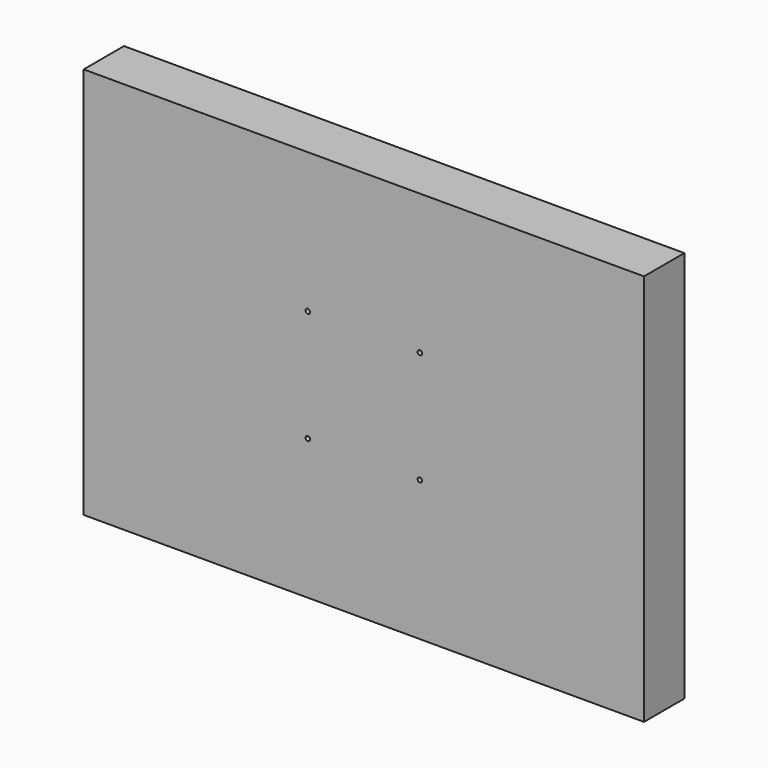
from build123d import *

# Parameters (mm, degrees)
F0_W     = 500
F0_H     = 350
F1_DEPTH = 50
F2_R     = 2
F3_DEPTH = 10
F4_W     = 400
F4_H     = 250
F5_DEPTH = 5
F6_SIZE  = 4.99999


# Not quite as in the source:
# - a fillet or chamfer is up to 0.001 mm smaller than in the source, because OpenCascade refuses the exact size


with BuildPart() as f1:
    # F0 (on Front) → F1 (new body)
    with BuildSketch(Plane.XZ):
        Rectangle(F0_W, F0_H)
    extrude(amount=F1_DEPTH)

    # F2 (on face) → F3 (cut)
    with BuildSketch(Plane.XZ.offset(50)):
        with Locations((-50, 50)):
            Circle(F2_R)
        with Locations((50, 50)):
            Circle(F2_R)
        with Locations((50, -50)):
            Circle(F2_R)
        with Locations((-50, -50)):
            Circle(F2_R)
    extrude(amount=-F3_DEPTH, mode=Mode.SUBTRACT)

    # F4 (on face) → F5 (cut)
    with BuildSketch(Plane(origin=(0, 0, 0), x_dir=(-1, 0, 0), z_dir=(0, 1, 0))):
        Rectangle(F4_W, F4_H)
    extrude(amount=-F5_DEPTH, mode=Mode.SUBTRACT)

    # F6 (size 5 in the source; OpenCascade refuses exactly that, so slightly less here)
    f6_edges = [f1.edges().sort_by_distance(p)[0] for p in [
        (250, 0, 0),
        (0, 0, -175),
        (0, 0, 175),
        (-250, 0, 0),
        (-200, 0, 0),
        (0, 0, -125),
        (200, 0, 0),
        (0, 0, 125),
    ]]
    chamfer(f6_edges, length=F6_SIZE)


solid = f1.part
